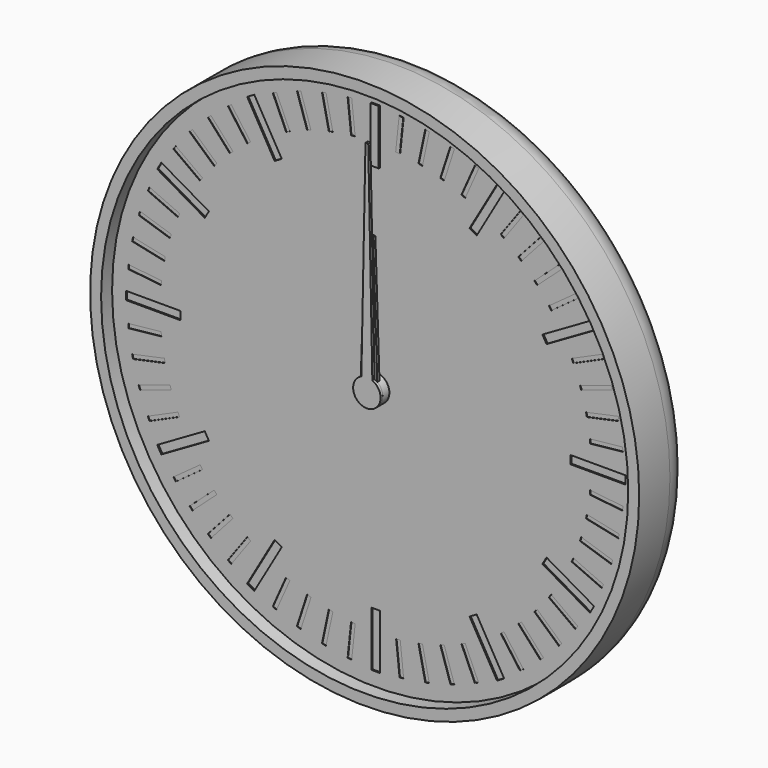
from build123d import *

# Parameters (mm, degrees)
F0_R      = 100
F1_DEPTH  = 24
F2_R      = 10
F3_T      = -4
F4_R      = 5
F4_R_2    = 3
F5_DEPTH  = 2
F6_DEPTH  = 19
F7_DEPTH  = 8
F9_DEPTH  = 4
F11_DEPTH = 4
F12_R     = 5
F12_R_2   = 3
F13_DEPTH = 2
F14_R     = 3
F15_DEPTH = 4
F17_DEPTH = 4
F18_R     = 3
F19_DEPTH = 2
F20_R     = 98
F20_R_2   = 5
F21_DEPTH = 1
F23_R     = 5
F23_R_2   = 3
F24_DEPTH = 2
F25_W     = 3
F25_H     = 20
F25_W_2   = 20
F25_H_2   = 3
F26_DEPTH = 0.5
F27_W     = 1.5
F27_H     = 12
F27_W_2   = 12
F27_H_2   = 1.5
F28_DEPTH = 0.2
F29_DEPTH = 1
F30_DEPTH = 0.4
F31_R     = 5
F31_R_2   = 3
F32_DEPTH = 5
F33_R     = 3
F34_DEPTH = 1
F36_DEPTH = 1


with BuildPart() as f1:
    # F0 (on Front) → F1 (new body)
    with BuildSketch(Plane.XZ):
        Circle(F0_R)
    extrude(amount=F1_DEPTH)

    # F2
    f2_edges = [f1.edges().sort_by_distance(p)[0] for p in [
        (-100, 0, 0),
    ]]
    fillet(f2_edges, radius=F2_R)

    # F3
    f3_openings = [f1.faces().sort_by_distance(p)[0] for p in [
        (0, -24, 0),
    ]]
    offset(amount=F3_T, openings=f3_openings)

    # F4 (on face) → F5 (join)
    with BuildSketch(Plane.XZ.offset(4)):
        Circle(F4_R)
        Circle(F4_R_2, mode=Mode.SUBTRACT)
        with Locations((40, 0)):
            Circle(F4_R)
        with Locations((40, 0)):
            Circle(F4_R_2, mode=Mode.SUBTRACT)
    extrude(amount=F5_DEPTH)


with BuildPart() as f6:
    # F6 (new): a face of the model
    f6_faces = [f1.part.faces().sort_by_distance(p)[0] for p in [
        (0, -4, 0),
    ]]
    extrude(f6_faces, amount=F6_DEPTH)

    # F8 (on face) → F9 (join)
    with BuildSketch(Plane.XZ.offset(6)):
        with BuildLine():
            ThreePointArc((9.2729637667, -1.3794085621), (9.3494561423, -0.6915886375), (9.375, 0))
            ThreePointArc((9.375, 0), (9.3494561423, 0.6915886375), (9.2729637667, 1.3794085621))
            ThreePointArc((9.2729637667, 1.3794085621), (8.9161548403, 2.8970343223), (8.3127812852, 4.3345463782))
            ThreePointArc((8.3127812852, 4.3345463782), (7.5845343223, 5.5104867402), (6.6911892658, 6.566476316))
            ThreePointArc((6.6911892658, 6.566476316), (5.5104867402, 7.5845343223), (4.1773988938, 8.3928519278))
            ThreePointArc((4.1773988938, 8.3928519278), (2.8970343223, 8.9161548403), (1.5536078905, 9.2453733036))
            ThreePointArc((1.5536078905, 9.2453733036), (0, 9.375), (-1.5536078905, 9.2453733036))
            ThreePointArc((-1.5536078905, 9.2453733036), (-2.8970343223, 8.9161548403), (-4.1773988938, 8.3928519278))
            ThreePointArc((-4.1773988938, 8.3928519278), (-5.5104867402, 7.5845343223), (-6.6911892658, 6.566476316))
            ThreePointArc((-6.6911892658, 6.566476316), (-7.5845343223, 5.5104867402), (-8.3127812852, 4.3345463782))
            ThreePointArc((-8.3127812852, 4.3345463782), (-8.9161548403, 2.8970343223), (-9.2729637667, 1.3794085621))
            ThreePointArc((-9.2729637667, 1.3794085621), (-9.375, 0), (-9.2729637667, -1.3794085621))
            ThreePointArc((-9.2729637667, -1.3794085621), (-8.9161548403, -2.8970343223), (-8.3127812852, -4.3345463782))
            ThreePointArc((-8.3127812852, -4.3345463782), (-7.5845343223, -5.5104867402), (-6.6911892658, -6.566476316))
            ThreePointArc((-6.6911892658, -6.566476316), (-5.5104867402, -7.5845343223), (-4.1773988938, -8.3928519278))
            ThreePointArc((-4.1773988938, -8.3928519278), (-2.8970343223, -8.9161548403), (-1.5536078905, -9.2453733036))
            ThreePointArc((-1.5536078905, -9.2453733036), (0, -9.375), (1.5536078905, -9.2453733036))
            ThreePointArc((1.5536078905, -9.2453733036), (2.8970343223, -8.9161548403), (4.1773988938, -8.3928519278))
            ThreePointArc((4.1773988938, -8.3928519278), (5.5104867402, -7.5845343223), (6.6911892658, -6.566476316))
            ThreePointArc((6.6911892658, -6.566476316), (7.5845343223, -5.5104867402), (8.3127812852, -4.3345463782))
            ThreePointArc((8.3127812852, -4.3345463782), (8.9161548403, -2.8970343223), (9.2729637667, -1.3794085621))
        make_face()
        with BuildLine():
            ThreePointArc((8.3127812852, 4.3345463782), (8.9161548403, 2.8970343223), (9.2729637667, 1.3794085621))
            Line((9.2729637667, 1.3794085621), (11.1823199426, 2.3946312492))
            Line((11.1823199426, 2.3946312492), (10.8182678729, 3.515068311))
            Line((10.8182678729, 3.515068311), (10.4542158031, 4.6355053728))
            Line((10.4542158031, 4.6355053728), (8.3127812852, 4.3345463782))
        make_face()
        with BuildLine():
            Line((11.1823199426, -2.3946312492), (9.2729637667, -1.3794085621))
            ThreePointArc((9.2729637667, -1.3794085621), (8.9161548403, -2.8970343223), (8.3127812852, -4.3345463782))
            Line((8.3127812852, -4.3345463782), (10.4542158031, -4.6355053728))
            Line((10.4542158031, -4.6355053728), (10.8182678729, -3.515068311))
            Line((10.8182678729, -3.515068311), (11.1823199426, -2.3946312492))
        make_face()
        with BuildLine():
            ThreePointArc((4.1773988938, 8.3928519278), (5.5104867402, 7.5845343223), (6.6911892658, 6.566476316))
            Line((6.6911892658, 6.566476316), (7.6391579371, 8.5101001246))
            Line((7.6391579371, 8.5101001246), (6.6860572448, 9.202568311))
            Line((6.6860572448, 9.202568311), (5.7329565525, 9.8950364974))
            Line((5.7329565525, 9.8950364974), (4.1773988938, 8.3928519278))
        make_face()
        with BuildLine():
            Line((7.6391579371, -8.5101001246), (6.6911892658, -6.566476316))
            ThreePointArc((6.6911892658, -6.566476316), (5.5104867402, -7.5845343223), (4.1773988938, -8.3928519278))
            Line((4.1773988938, -8.3928519278), (5.7329565525, -9.8950364974))
            Line((5.7329565525, -9.8950364974), (6.6860572448, -9.202568311))
            Line((6.6860572448, -9.202568311), (7.6391579371, -8.5101001246))
        make_face()
        with BuildLine():
            ThreePointArc((-1.5536078905, 9.2453733036), (0, 9.375), (1.5536078905, 9.2453733036))
            Line((1.5536078905, 9.2453733036), (1.1780972451, 11.375))
            Line((1.1780972451, 11.375), (0, 11.375))
            Line((0, 11.375), (-1.1780972451, 11.375))
            Line((-1.1780972451, 11.375), (-1.5536078905, 9.2453733036))
        make_face()
        with BuildLine():
            Line((1.1780972451, -11.375), (1.5536078905, -9.2453733036))
            ThreePointArc((1.5536078905, -9.2453733036), (0, -9.375), (-1.5536078905, -9.2453733036))
            Line((-1.5536078905, -9.2453733036), (-1.1780972451, -11.375))
            Line((-1.1780972451, -11.375), (0, -11.375))
            Line((0, -11.375), (1.1780972451, -11.375))
        make_face()
        with BuildLine():
            ThreePointArc((-6.6911892658, 6.566476316), (-5.5104867402, 7.5845343223), (-4.1773988938, 8.3928519278))
            Line((-4.1773988938, 8.3928519278), (-5.7329565525, 9.8950364974))
            Line((-5.7329565525, 9.8950364974), (-6.6860572448, 9.202568311))
            Line((-6.6860572448, 9.202568311), (-7.6391579371, 8.5101001246))
            Line((-7.6391579371, 8.5101001246), (-6.6911892658, 6.566476316))
        make_face()
        with BuildLine():
            Line((-5.7329565525, -9.8950364974), (-4.1773988938, -8.3928519278))
            ThreePointArc((-4.1773988938, -8.3928519278), (-5.5104867402, -7.5845343223), (-6.6911892658, -6.566476316))
            Line((-6.6911892658, -6.566476316), (-7.6391579371, -8.5101001246))
            Line((-7.6391579371, -8.5101001246), (-6.6860572448, -9.202568311))
            Line((-6.6860572448, -9.202568311), (-5.7329565525, -9.8950364974))
        make_face()
        with BuildLine():
            ThreePointArc((-9.2729637667, 1.3794085621), (-8.9161548403, 2.8970343223), (-8.3127812852, 4.3345463782))
            Line((-8.3127812852, 4.3345463782), (-10.4542158031, 4.6355053728))
            Line((-10.4542158031, 4.6355053728), (-10.8182678729, 3.515068311))
            Line((-10.8182678729, 3.515068311), (-11.1823199426, 2.3946312492))
            Line((-11.1823199426, 2.3946312492), (-9.2729637667, 1.3794085621))
        make_face()
        with BuildLine():
            Line((-10.4542158031, -4.6355053728), (-8.3127812852, -4.3345463782))
            ThreePointArc((-8.3127812852, -4.3345463782), (-8.9161548403, -2.8970343223), (-9.2729637667, -1.3794085621))
            Line((-9.2729637667, -1.3794085621), (-11.1823199426, -2.3946312492))
            Line((-11.1823199426, -2.3946312492), (-10.8182678729, -3.515068311))
            Line((-10.8182678729, -3.515068311), (-10.4542158031, -4.6355053728))
        make_face()
    extrude(amount=F9_DEPTH)

    # F35 (on face) → F36 (join)
    with BuildSketch(Plane.XZ.offset(23)):
        with BuildLine():
            ThreePointArc((-2, 4.582575695), (-2.7386127875, -4.1833001327), (5, 0))
            ThreePointArc((5, 0), (4.1833001327, 2.7386127875), (2, 4.582575695))
            ThreePointArc((2, 4.582575695), (0, 5), (-2, 4.582575695))
        make_face()
        with BuildLine():
            ThreePointArc((-2, 4.582575695), (0, 5), (2, 4.582575695))
            Line((2, 4.582575695), (0.5, 80))
            Line((0.5, 80), (0, 80))
            Line((0, 80), (-0.5, 80))
            Line((-0.5, 80), (-2, 4.582575695))
        make_face()
    extrude(amount=-F36_DEPTH)


with BuildPart() as f7:
    # F7 (new): a face of the model
    f7_faces = [f1.part.faces().sort_by_distance(p)[0] for p in [
        (40, -4, 0),
    ]]
    extrude(f7_faces, amount=F7_DEPTH)

    # F10 (on face) → F11 (join)
    with BuildSketch(Plane.XZ.offset(6)):
        with BuildLine():
            ThreePointArc((68.0829066802, -1.5381733945), (68.1144747006, -0.7693746225), (68.125, 0))
            ThreePointArc((68.125, 0), (68.1144747006, 0.7693746225), (68.0829066802, 1.5381733945))
            ThreePointArc((68.0829066802, 1.5381733945), (67.9709283072, 2.9398630294), (67.7890320221, 4.3342039956))
            ThreePointArc((67.7890320221, 4.3342039956), (67.5104012706, 5.8475163042), (67.1494235596, 7.3433252263))
            ThreePointArc((67.1494235596, 7.3433252263), (66.7484645208, 8.6911029668), (66.280643318, 10.0171558733))
            ThreePointArc((66.280643318, 10.0171558733), (65.6934659962, 11.4394680865), (65.0293803521, 12.8275385085))
            ThreePointArc((65.0293803521, 12.8275385085), (64.3569644814, 14.0625), (63.6236643925, 15.2623099717))
            ThreePointArc((63.6236643925, 15.2623099717), (62.7536029668, 16.5314602207), (61.815433119, 17.7511268046))
            ThreePointArc((61.815433119, 17.7511268046), (60.9009482166, 18.8192983038), (59.934217974, 19.8404278876))
            ThreePointArc((59.934217974, 19.8404278876), (58.8192983038, 20.9009482166), (57.6480467764, 21.8989056799))
            ThreePointArc((57.6480467764, 21.8989056799), (56.5314602207, 22.7536029668), (55.3735505752, 23.5514238999))
            ThreePointArc((55.3735505752, 23.5514238999), (54.0625, 24.3569644814), (52.709356105, 25.0895972944))
            ThreePointArc((52.709356105, 25.0895972944), (51.4394680865, 25.6934659962), (50.1409852457, 26.2331096755))
            ThreePointArc((50.1409852457, 26.2331096755), (48.6911029668, 26.7484645208), (47.2152055856, 27.1837531139))
            ThreePointArc((47.2152055856, 27.1837531139), (45.8475163042, 27.5104012706), (44.4652101991, 27.7682826779))
            ThreePointArc((44.4652101991, 27.7682826779), (42.9398630294, 27.9709283072), (41.4057159597, 28.0898484802))
            ThreePointArc((41.4057159597, 28.0898484802), (40, 28.125), (38.5942840403, 28.0898484802))
            ThreePointArc((38.5942840403, 28.0898484802), (37.0601369706, 27.9709283072), (35.5347898009, 27.7682826779))
            ThreePointArc((35.5347898009, 27.7682826779), (34.1524836958, 27.5104012706), (32.7847944144, 27.1837531139))
            ThreePointArc((32.7847944144, 27.1837531139), (31.3088970332, 26.7484645208), (29.8590147543, 26.2331096755))
            ThreePointArc((29.8590147543, 26.2331096755), (28.5605319135, 25.6934659962), (27.290643895, 25.0895972944))
            ThreePointArc((27.290643895, 25.0895972944), (25.9375, 24.3569644814), (24.6264494248, 23.5514238999))
            ThreePointArc((24.6264494248, 23.5514238999), (23.4685397793, 22.7536029668), (22.3519532236, 21.8989056799))
            ThreePointArc((22.3519532236, 21.8989056799), (21.1807016962, 20.9009482166), (20.065782026, 19.8404278876))
            ThreePointArc((20.065782026, 19.8404278876), (19.0990517834, 18.8192983038), (18.184566881, 17.7511268046))
            ThreePointArc((18.184566881, 17.7511268046), (17.2463970332, 16.5314602207), (16.3763356075, 15.2623099717))
            ThreePointArc((16.3763356075, 15.2623099717), (15.6430355186, 14.0625), (14.9706196479, 12.8275385085))
            ThreePointArc((14.9706196479, 12.8275385085), (14.3065340038, 11.4394680865), (13.719356682, 10.0171558733))
            ThreePointArc((13.719356682, 10.0171558733), (13.2515354792, 8.6911029668), (12.8505764404, 7.3433252263))
            ThreePointArc((12.8505764404, 7.3433252263), (12.4895987294, 5.8475163042), (12.2109679779, 4.3342039956))
            ThreePointArc((12.2109679779, 4.3342039956), (12.0290716928, 2.9398630294), (11.9170933198, 1.5381733945))
            ThreePointArc((11.9170933198, 1.5381733945), (11.875, 0), (11.9170933198, -1.5381733945))
            ThreePointArc((11.9170933198, -1.5381733945), (12.0290716928, -2.9398630294), (12.2109679779, -4.3342039956))
            ThreePointArc((12.2109679779, -4.3342039956), (12.4895987294, -5.8475163042), (12.8505764404, -7.3433252263))
            ThreePointArc((12.8505764404, -7.3433252263), (13.2515354792, -8.6911029668), (13.719356682, -10.0171558733))
            ThreePointArc((13.719356682, -10.0171558733), (14.3065340038, -11.4394680865), (14.9706196479, -12.8275385085))
            ThreePointArc((14.9706196479, -12.8275385085), (15.6430355186, -14.0625), (16.3763356075, -15.2623099717))
            ThreePointArc((16.3763356075, -15.2623099717), (17.2463970332, -16.5314602207), (18.184566881, -17.7511268046))
            ThreePointArc((18.184566881, -17.7511268046), (19.0990517834, -18.8192983038), (20.065782026, -19.8404278876))
            ThreePointArc((20.065782026, -19.8404278876), (21.1807016962, -20.9009482166), (22.3519532236, -21.8989056799))
            ThreePointArc((22.3519532236, -21.8989056799), (23.4685397793, -22.7536029668), (24.6264494248, -23.5514238999))
            ThreePointArc((24.6264494248, -23.5514238999), (25.9375, -24.3569644814), (27.290643895, -25.0895972944))
            ThreePointArc((27.290643895, -25.0895972944), (28.5605319135, -25.6934659962), (29.8590147543, -26.2331096755))
            ThreePointArc((29.8590147543, -26.2331096755), (31.3088970332, -26.7484645208), (32.7847944144, -27.1837531139))
            ThreePointArc((32.7847944144, -27.1837531139), (34.1524836958, -27.5104012706), (35.5347898009, -27.7682826779))
            ThreePointArc((35.5347898009, -27.7682826779), (37.0601369706, -27.9709283072), (38.5942840403, -28.0898484802))
            ThreePointArc((38.5942840403, -28.0898484802), (40, -28.125), (41.4057159597, -28.0898484802))
            ThreePointArc((41.4057159597, -28.0898484802), (42.9398630294, -27.9709283072), (44.4652101991, -27.7682826779))
            ThreePointArc((44.4652101991, -27.7682826779), (45.8475163042, -27.5104012706), (47.2152055856, -27.1837531139))
            ThreePointArc((47.2152055856, -27.1837531139), (48.6911029668, -26.7484645208), (50.1409852457, -26.2331096755))
            ThreePointArc((50.1409852457, -26.2331096755), (51.4394680865, -25.6934659962), (52.709356105, -25.0895972944))
            ThreePointArc((52.709356105, -25.0895972944), (54.0625, -24.3569644814), (55.3735505752, -23.5514238999))
            ThreePointArc((55.3735505752, -23.5514238999), (56.5314602207, -22.7536029668), (57.6480467764, -21.8989056799))
            ThreePointArc((57.6480467764, -21.8989056799), (58.8192983038, -20.9009482166), (59.934217974, -19.8404278876))
            ThreePointArc((59.934217974, -19.8404278876), (60.9009482166, -18.8192983038), (61.815433119, -17.7511268046))
            ThreePointArc((61.815433119, -17.7511268046), (62.7536029668, -16.5314602207), (63.6236643925, -15.2623099717))
            ThreePointArc((63.6236643925, -15.2623099717), (64.3569644814, -14.0625), (65.0293803521, -12.8275385085))
            ThreePointArc((65.0293803521, -12.8275385085), (65.6934659962, -11.4394680865), (66.280643318, -10.0171558733))
            ThreePointArc((66.280643318, -10.0171558733), (66.7484645208, -8.6911029668), (67.1494235596, -7.3433252263))
            ThreePointArc((67.1494235596, -7.3433252263), (67.5104012706, -5.8475163042), (67.7890320221, -4.3342039956))
            ThreePointArc((67.7890320221, -4.3342039956), (67.9709283072, -2.9398630294), (68.0829066802, -1.5381733945))
        make_face()
        with BuildLine():
            ThreePointArc((68.0829066802, 1.5381733945), (68.1144747006, 0.7693746225), (68.125, 0))
            ThreePointArc((68.125, 0), (68.1144747006, -0.7693746225), (68.0829066802, -1.5381733945))
            Line((68.0829066802, -1.5381733945), (70.125, -1.1780972451))
            Line((70.125, -1.1780972451), (70.125, 0))
            Line((70.125, 0), (70.125, 1.1780972451))
            Line((70.125, 1.1780972451), (68.0829066802, 1.5381733945))
        make_face()
        with BuildLine():
            ThreePointArc((67.1494235596, 7.3433252263), (67.5104012706, 5.8475163042), (67.7890320221, 4.3342039956))
            Line((67.7890320221, 4.3342039956), (69.7116366623, 5.1109866922))
            Line((69.7116366623, 5.1109866922), (69.4666964721, 6.2633396859))
            Line((69.4666964721, 6.2633396859), (69.2217562819, 7.4156926796))
            Line((69.2217562819, 7.4156926796), (67.1494235596, 7.3433252263))
        make_face()
        with BuildLine():
            Line((69.7116366623, -5.1109866922), (67.7890320221, -4.3342039956))
            ThreePointArc((67.7890320221, -4.3342039956), (67.5104012706, -5.8475163042), (67.1494235596, -7.3433252263))
            Line((67.1494235596, -7.3433252263), (69.2217562819, -7.4156926796))
            Line((69.2217562819, -7.4156926796), (69.4666964721, -6.2633396859))
            Line((69.4666964721, -6.2633396859), (69.7116366623, -5.1109866922))
        make_face()
        with BuildLine():
            ThreePointArc((65.0293803521, 12.8275385085), (65.6934659962, 11.4394680865), (66.280643318, 10.0171558733))
            Line((66.280643318, 10.0171558733), (67.9997322302, 11.1766959857))
            Line((67.9997322302, 11.1766959857), (67.5205569115, 12.2529413727))
            Line((67.5205569115, 12.2529413727), (67.0413815928, 13.3291867596))
            Line((67.0413815928, 13.3291867596), (65.0293803521, 12.8275385085))
        make_face()
        with BuildLine():
            Line((67.9997322302, -11.1766959857), (66.280643318, -10.0171558733))
            ThreePointArc((66.280643318, -10.0171558733), (65.6934659962, -11.4394680865), (65.0293803521, -12.8275385085))
            Line((65.0293803521, -12.8275385085), (67.0413815928, -13.3291867596))
            Line((67.0413815928, -13.3291867596), (67.5205569115, -12.2529413727))
            Line((67.5205569115, -12.2529413727), (67.9997322302, -11.1766959857))
        make_face()
        with BuildLine():
            ThreePointArc((61.815433119, 17.7511268046), (62.7536029668, 16.5314602207), (63.6236643925, 15.2623099717))
            Line((63.6236643925, 15.2623099717), (65.064105142, 16.753930033))
            Line((65.064105142, 16.753930033), (64.3716369555, 17.7070307253))
            Line((64.3716369555, 17.7070307253), (63.6791687691, 18.6601314176))
            Line((63.6791687691, 18.6601314176), (61.815433119, 17.7511268046))
        make_face()
        with BuildLine():
            Line((65.064105142, -16.753930033), (63.6236643925, -15.2623099717))
            ThreePointArc((63.6236643925, -15.2623099717), (62.7536029668, -16.5314602207), (61.815433119, -17.7511268046))
            Line((61.815433119, -17.7511268046), (63.6791687691, -18.6601314176))
            Line((63.6791687691, -18.6601314176), (64.3716369555, -17.7070307253))
            Line((64.3716369555, -17.7070307253), (65.064105142, -16.753930033))
        make_face()
        with BuildLine():
            ThreePointArc((57.6480467764, 21.8989056799), (58.8192983038, 20.9009482166), (59.934217974, 19.8404278876))
            Line((59.934217974, 19.8404278876), (61.0330563882, 21.5989369435))
            Line((61.0330563882, 21.5989369435), (60.1575595166, 22.3872378675))
            Line((60.1575595166, 22.3872378675), (59.282062645, 23.1755387915))
            Line((59.282062645, 23.1755387915), (57.6480467764, 21.8989056799))
        make_face()
        with BuildLine():
            Line((61.0330563882, -21.5989369435), (59.934217974, -19.8404278876))
            ThreePointArc((59.934217974, -19.8404278876), (58.8192983038, -20.9009482166), (57.6480467764, -21.8989056799))
            Line((57.6480467764, -21.8989056799), (59.282062645, -23.1755387915))
            Line((59.282062645, -23.1755387915), (60.1575595166, -22.3872378675))
            Line((60.1575595166, -22.3872378675), (61.0330563882, -21.5989369435))
        make_face()
        with BuildLine():
            ThreePointArc((52.709356105, 25.0895972944), (54.0625, 24.3569644814), (55.3735505752, 23.5514238999))
            Line((55.3735505752, 23.5514238999), (56.0827621424, 25.4999666665))
            Line((56.0827621424, 25.4999666665), (55.0625, 26.089015289))
            Line((55.0625, 26.089015289), (54.0422378576, 26.6780639116))
            Line((54.0422378576, 26.6780639116), (52.709356105, 25.0895972944))
        make_face()
        with BuildLine():
            Line((56.0827621424, -25.4999666665), (55.3735505752, -23.5514238999))
            ThreePointArc((55.3735505752, -23.5514238999), (54.0625, -24.3569644814), (52.709356105, -25.0895972944))
            Line((52.709356105, -25.0895972944), (54.0422378576, -26.6780639116))
            Line((54.0422378576, -26.6780639116), (55.0625, -26.089015289))
            Line((55.0625, -26.089015289), (56.0827621424, -25.4999666665))
        make_face()
        with BuildLine():
            ThreePointArc((47.2152055856, 27.1837531139), (48.6911029668, 26.7484645208), (50.1409852457, 26.2331096755))
            Line((50.1409852457, 26.2331096755), (50.4295740173, 28.2865254836))
            Line((50.4295740173, 28.2865254836), (49.3091369555, 28.6505775534))
            Line((49.3091369555, 28.6505775534), (48.1886998938, 29.0146296232))
            Line((48.1886998938, 29.0146296232), (47.2152055856, 27.1837531139))
        make_face()
        with BuildLine():
            Line((50.4295740173, -28.2865254836), (50.1409852457, -26.2331096755))
            ThreePointArc((50.1409852457, -26.2331096755), (48.6911029668, -26.7484645208), (47.2152055856, -27.1837531139))
            Line((47.2152055856, -27.1837531139), (48.1886998938, -29.0146296232))
            Line((48.1886998938, -29.0146296232), (49.3091369555, -28.6505775534))
            Line((49.3091369555, -28.6505775534), (50.4295740173, -28.2865254836))
        make_face()
        with BuildLine():
            ThreePointArc((41.4057159597, 28.0898484802), (42.9398630294, 27.9709283072), (44.4652101991, 27.7682826779))
            Line((44.4652101991, 27.7682826779), (44.3205634611, 29.8368274034))
            Line((44.3205634611, 29.8368274034), (43.1489199559, 29.959972098))
            Line((43.1489199559, 29.959972098), (41.9772764508, 30.0831167926))
            Line((41.9772764508, 30.0831167926), (41.4057159597, 28.0898484802))
        make_face()
        with BuildLine():
            Line((44.3205634611, -29.8368274034), (44.4652101991, -27.7682826779))
            ThreePointArc((44.4652101991, -27.7682826779), (42.9398630294, -27.9709283072), (41.4057159597, -28.0898484802))
            Line((41.4057159597, -28.0898484802), (41.9772764508, -30.0831167926))
            Line((41.9772764508, -30.0831167926), (43.1489199559, -29.959972098))
            Line((43.1489199559, -29.959972098), (44.3205634611, -29.8368274034))
        make_face()
        with BuildLine():
            ThreePointArc((35.5347898009, 27.7682826779), (37.0601369706, 27.9709283072), (38.5942840403, 28.0898484802))
            Line((38.5942840403, 28.0898484802), (38.0227235492, 30.0831167926))
            Line((38.0227235492, 30.0831167926), (36.8510800441, 29.959972098))
            Line((36.8510800441, 29.959972098), (35.6794365389, 29.8368274034))
            Line((35.6794365389, 29.8368274034), (35.5347898009, 27.7682826779))
        make_face()
        with BuildLine():
            Line((38.0227235492, -30.0831167926), (38.5942840403, -28.0898484802))
            ThreePointArc((38.5942840403, -28.0898484802), (37.0601369706, -27.9709283072), (35.5347898009, -27.7682826779))
            Line((35.5347898009, -27.7682826779), (35.6794365389, -29.8368274034))
            Line((35.6794365389, -29.8368274034), (36.8510800441, -29.959972098))
            Line((36.8510800441, -29.959972098), (38.0227235492, -30.0831167926))
        make_face()
        with BuildLine():
            ThreePointArc((29.8590147543, 26.2331096755), (31.3088970332, 26.7484645208), (32.7847944144, 27.1837531139))
            Line((32.7847944144, 27.1837531139), (31.8113001062, 29.0146296232))
            Line((31.8113001062, 29.0146296232), (30.6908630445, 28.6505775534))
            Line((30.6908630445, 28.6505775534), (29.5704259827, 28.2865254836))
            Line((29.5704259827, 28.2865254836), (29.8590147543, 26.2331096755))
        make_face()
        with BuildLine():
            Line((31.8113001062, -29.0146296232), (32.7847944144, -27.1837531139))
            ThreePointArc((32.7847944144, -27.1837531139), (31.3088970332, -26.7484645208), (29.8590147543, -26.2331096755))
            Line((29.8590147543, -26.2331096755), (29.5704259827, -28.2865254836))
            Line((29.5704259827, -28.2865254836), (30.6908630445, -28.6505775534))
            Line((30.6908630445, -28.6505775534), (31.8113001062, -29.0146296232))
        make_face()
        with BuildLine():
            ThreePointArc((24.6264494248, 23.5514238999), (25.9375, 24.3569644814), (27.290643895, 25.0895972944))
            Line((27.290643895, 25.0895972944), (25.9577621424, 26.6780639116))
            Line((25.9577621424, 26.6780639116), (24.9375, 26.089015289))
            Line((24.9375, 26.089015289), (23.9172378576, 25.4999666665))
            Line((23.9172378576, 25.4999666665), (24.6264494248, 23.5514238999))
        make_face()
        with BuildLine():
            Line((25.9577621424, -26.6780639116), (27.290643895, -25.0895972944))
            ThreePointArc((27.290643895, -25.0895972944), (25.9375, -24.3569644814), (24.6264494248, -23.5514238999))
            Line((24.6264494248, -23.5514238999), (23.9172378576, -25.4999666665))
            Line((23.9172378576, -25.4999666665), (24.9375, -26.089015289))
            Line((24.9375, -26.089015289), (25.9577621424, -26.6780639116))
        make_face()
        with BuildLine():
            ThreePointArc((20.065782026, 19.8404278876), (21.1807016962, 20.9009482166), (22.3519532236, 21.8989056799))
            Line((22.3519532236, 21.8989056799), (20.717937355, 23.1755387915))
            Line((20.717937355, 23.1755387915), (19.8424404834, 22.3872378675))
            Line((19.8424404834, 22.3872378675), (18.9669436118, 21.5989369435))
            Line((18.9669436118, 21.5989369435), (20.065782026, 19.8404278876))
        make_face()
        with BuildLine():
            Line((20.717937355, -23.1755387915), (22.3519532236, -21.8989056799))
            ThreePointArc((22.3519532236, -21.8989056799), (21.1807016962, -20.9009482166), (20.065782026, -19.8404278876))
            Line((20.065782026, -19.8404278876), (18.9669436118, -21.5989369435))
            Line((18.9669436118, -21.5989369435), (19.8424404834, -22.3872378675))
            Line((19.8424404834, -22.3872378675), (20.717937355, -23.1755387915))
        make_face()
        with BuildLine():
            ThreePointArc((16.3763356075, 15.2623099717), (17.2463970332, 16.5314602207), (18.184566881, 17.7511268046))
            Line((18.184566881, 17.7511268046), (16.3208312309, 18.6601314176))
            Line((16.3208312309, 18.6601314176), (15.6283630445, 17.7070307253))
            Line((15.6283630445, 17.7070307253), (14.935894858, 16.753930033))
            Line((14.935894858, 16.753930033), (16.3763356075, 15.2623099717))
        make_face()
        with BuildLine():
            Line((16.3208312309, -18.6601314176), (18.184566881, -17.7511268046))
            ThreePointArc((18.184566881, -17.7511268046), (17.2463970332, -16.5314602207), (16.3763356075, -15.2623099717))
            Line((16.3763356075, -15.2623099717), (14.935894858, -16.753930033))
            Line((14.935894858, -16.753930033), (15.6283630445, -17.7070307253))
            Line((15.6283630445, -17.7070307253), (16.3208312309, -18.6601314176))
        make_face()
        with BuildLine():
            ThreePointArc((13.719356682, 10.0171558733), (14.3065340038, 11.4394680865), (14.9706196479, 12.8275385085))
            Line((14.9706196479, 12.8275385085), (12.9586184072, 13.3291867596))
            Line((12.9586184072, 13.3291867596), (12.4794430885, 12.2529413727))
            Line((12.4794430885, 12.2529413727), (12.0002677698, 11.1766959857))
            Line((12.0002677698, 11.1766959857), (13.719356682, 10.0171558733))
        make_face()
        with BuildLine():
            Line((12.9586184072, -13.3291867596), (14.9706196479, -12.8275385085))
            ThreePointArc((14.9706196479, -12.8275385085), (14.3065340038, -11.4394680865), (13.719356682, -10.0171558733))
            Line((13.719356682, -10.0171558733), (12.0002677698, -11.1766959857))
            Line((12.0002677698, -11.1766959857), (12.4794430885, -12.2529413727))
            Line((12.4794430885, -12.2529413727), (12.9586184072, -13.3291867596))
        make_face()
        with BuildLine():
            ThreePointArc((12.2109679779, 4.3342039956), (12.4895987294, 5.8475163042), (12.8505764404, 7.3433252263))
            Line((12.8505764404, 7.3433252263), (10.7782437181, 7.4156926796))
            Line((10.7782437181, 7.4156926796), (10.5333035279, 6.2633396859))
            Line((10.5333035279, 6.2633396859), (10.2883633377, 5.1109866922))
            Line((10.2883633377, 5.1109866922), (12.2109679779, 4.3342039956))
        make_face()
        with BuildLine():
            Line((10.7782437181, -7.4156926796), (12.8505764404, -7.3433252263))
            ThreePointArc((12.8505764404, -7.3433252263), (12.4895987294, -5.8475163042), (12.2109679779, -4.3342039956))
            Line((12.2109679779, -4.3342039956), (10.2883633377, -5.1109866922))
            Line((10.2883633377, -5.1109866922), (10.5333035279, -6.2633396859))
            Line((10.5333035279, -6.2633396859), (10.7782437181, -7.4156926796))
        make_face()
        with BuildLine():
            ThreePointArc((11.9170933198, -1.5381733945), (11.875, 0), (11.9170933198, 1.5381733945))
            Line((11.9170933198, 1.5381733945), (9.875, 1.1780972451))
            Line((9.875, 1.1780972451), (9.875, 0))
            Line((9.875, 0), (9.875, -1.1780972451))
            Line((9.875, -1.1780972451), (11.9170933198, -1.5381733945))
        make_face()
    extrude(amount=F11_DEPTH)

    # F16 (on face) → F17 (join)
    with BuildSketch(Plane.XZ.offset(12)):
        with BuildLine():
            ThreePointArc((47.4288750323, -1.0304444454), (47.4821976298, -0.5164480894), (47.5, 0))
            ThreePointArc((47.5, 0), (47.4821976298, 0.5164480894), (47.4288750323, 1.0304444454))
            ThreePointArc((47.4288750323, 1.0304444454), (47.1329238722, 2.3176274578), (46.6157661985, 3.532936117))
            ThreePointArc((46.6157661985, 3.532936117), (46.0676274578, 4.4083893922), (45.4044061018, 5.2002302532))
            ThreePointArc((45.4044061018, 5.2002302532), (44.4083893922, 6.0676274578), (43.2756595386, 6.7468551628))
            ThreePointArc((43.2756595386, 6.7468551628), (42.3176274578, 7.1329238722), (41.3156377295, 7.3837048536))
            ThreePointArc((41.3156377295, 7.3837048536), (40, 7.5), (38.6843622705, 7.3837048536))
            ThreePointArc((38.6843622705, 7.3837048536), (37.6823725422, 7.1329238722), (36.7243404614, 6.7468551628))
            ThreePointArc((36.7243404614, 6.7468551628), (35.5916106078, 6.0676274578), (34.5955938982, 5.2002302532))
            ThreePointArc((34.5955938982, 5.2002302532), (33.9323725422, 4.4083893922), (33.3842338015, 3.532936117))
            ThreePointArc((33.3842338015, 3.532936117), (32.8670761278, 2.3176274578), (32.5711249677, 1.0304444454))
            ThreePointArc((32.5711249677, 1.0304444454), (32.5, 0), (32.5711249677, -1.0304444454))
            ThreePointArc((32.5711249677, -1.0304444454), (32.8670761278, -2.3176274578), (33.3842338015, -3.532936117))
            ThreePointArc((33.3842338015, -3.532936117), (33.9323725422, -4.4083893922), (34.5955938982, -5.2002302532))
            ThreePointArc((34.5955938982, -5.2002302532), (35.5916106078, -6.0676274578), (36.7243404614, -6.7468551628))
            ThreePointArc((36.7243404614, -6.7468551628), (37.6823725422, -7.1329238722), (38.6843622705, -7.3837048536))
            ThreePointArc((38.6843622705, -7.3837048536), (40, -7.5), (41.3156377295, -7.3837048536))
            ThreePointArc((41.3156377295, -7.3837048536), (42.3176274578, -7.1329238722), (43.2756595386, -6.7468551628))
            ThreePointArc((43.2756595386, -6.7468551628), (44.4083893922, -6.0676274578), (45.4044061018, -5.2002302532))
            ThreePointArc((45.4044061018, -5.2002302532), (46.0676274578, -4.4083893922), (46.6157661985, -3.532936117))
            ThreePointArc((46.6157661985, -3.532936117), (47.1329238722, -2.3176274578), (47.4288750323, -1.0304444454))
        make_face()
        with BuildLine():
            ThreePointArc((46.6157661985, 3.532936117), (47.1329238722, 2.3176274578), (47.4288750323, 1.0304444454))
            Line((47.4288750323, 1.0304444454), (49.3262785606, 2.0393117971))
            Line((49.3262785606, 2.0393117971), (48.743795249, 3.832011096))
            Line((48.743795249, 3.832011096), (46.6157661985, 3.532936117))
        make_face()
        with BuildLine():
            Line((49.3262785606, -2.0393117971), (47.4288750323, -1.0304444454))
            ThreePointArc((47.4288750323, -1.0304444454), (47.1329238722, -2.3176274578), (46.6157661985, -3.532936117))
            Line((46.6157661985, -3.532936117), (48.743795249, -3.832011096))
            Line((48.743795249, -3.832011096), (49.3262785606, -2.0393117971))
        make_face()
        with BuildLine():
            ThreePointArc((43.2756595386, 6.7468551628), (44.4083893922, 6.0676274578), (45.4044061018, 5.2002302532))
            Line((45.4044061018, 5.2002302532), (46.3464404506, 7.1316868974))
            Line((46.3464404506, 7.1316868974), (44.8214793429, 8.2396359957))
            Line((44.8214793429, 8.2396359957), (43.2756595386, 6.7468551628))
        make_face()
        with BuildLine():
            Line((46.3464404506, -7.1316868974), (45.4044061018, -5.2002302532))
            ThreePointArc((45.4044061018, -5.2002302532), (44.4083893922, -6.0676274578), (43.2756595386, -6.7468551628))
            Line((43.2756595386, -6.7468551628), (44.8214793429, -8.2396359957))
            Line((44.8214793429, -8.2396359957), (46.3464404506, -7.1316868974))
        make_face()
        with BuildLine():
            ThreePointArc((38.6843622705, 7.3837048536), (40, 7.5), (41.3156377295, 7.3837048536))
            Line((41.3156377295, 7.3837048536), (40.9424777961, 9.5))
            Line((40.9424777961, 9.5), (39.0575222039, 9.5))
            Line((39.0575222039, 9.5), (38.6843622705, 7.3837048536))
        make_face()
        with BuildLine():
            Line((40.9424777961, -9.5), (41.3156377295, -7.3837048536))
            ThreePointArc((41.3156377295, -7.3837048536), (40, -7.5), (38.6843622705, -7.3837048536))
            Line((38.6843622705, -7.3837048536), (39.0575222039, -9.5))
            Line((39.0575222039, -9.5), (40.9424777961, -9.5))
        make_face()
        with BuildLine():
            ThreePointArc((34.5955938982, 5.2002302532), (35.5916106078, 6.0676274578), (36.7243404614, 6.7468551628))
            Line((36.7243404614, 6.7468551628), (35.1785206571, 8.2396359957))
            Line((35.1785206571, 8.2396359957), (33.6535595494, 7.1316868974))
            Line((33.6535595494, 7.1316868974), (34.5955938982, 5.2002302532))
        make_face()
        with BuildLine():
            Line((35.1785206571, -8.2396359957), (36.7243404614, -6.7468551628))
            ThreePointArc((36.7243404614, -6.7468551628), (35.5916106078, -6.0676274578), (34.5955938982, -5.2002302532))
            Line((34.5955938982, -5.2002302532), (33.6535595494, -7.1316868974))
            Line((33.6535595494, -7.1316868974), (35.1785206571, -8.2396359957))
        make_face()
        with BuildLine():
            ThreePointArc((32.5711249677, 1.0304444454), (32.8670761278, 2.3176274578), (33.3842338015, 3.532936117))
            Line((33.3842338015, 3.532936117), (31.256204751, 3.832011096))
            Line((31.256204751, 3.832011096), (30.6737214394, 2.0393117971))
            Line((30.6737214394, 2.0393117971), (32.5711249677, 1.0304444454))
        make_face()
        with BuildLine():
            Line((31.256204751, -3.832011096), (33.3842338015, -3.532936117))
            ThreePointArc((33.3842338015, -3.532936117), (32.8670761278, -2.3176274578), (32.5711249677, -1.0304444454))
            Line((32.5711249677, -1.0304444454), (30.6737214394, -2.0393117971))
            Line((30.6737214394, -2.0393117971), (31.256204751, -3.832011096))
        make_face()
    extrude(amount=F17_DEPTH)

    # F18 (on face) → F19 (join)
    with BuildSketch(Plane.XZ.offset(16)):
        with Locations((40, 0)):
            Circle(F18_R)
    extrude(amount=F19_DEPTH)


with BuildPart() as f13:
    # F12 (on face) → F13 (new body)
    with BuildSketch(Plane.XZ.offset(10)):
        Circle(F12_R)
        Circle(F12_R_2, mode=Mode.SUBTRACT)
    extrude(amount=F13_DEPTH)

    # F14 (on face) → F15 (join)
    with BuildSketch(Plane.XZ.offset(12)):
        with BuildLine():
            ThreePointArc((29.9718156995, -1.3001014101), (29.9929530972, -0.6502034357), (30, 0))
            ThreePointArc((30, 0), (29.9929530972, 0.6502034357), (29.9718156995, 1.3001014101))
            ThreePointArc((29.9718156995, 1.3001014101), (29.907520012, 2.3537728718), (29.8061935814, 3.4045299509))
            ThreePointArc((29.8061935814, 3.4045299509), (29.6306502179, 4.6930339512), (29.3994322443, 5.9727199596))
            ThreePointArc((29.3994322443, 5.9727199596), (29.1710976119, 7.0033609157), (28.9066440563, 8.0253304855))
            ThreePointArc((28.9066440563, 8.0253304855), (28.5316954889, 9.2705098312), (28.1031371961, 10.4982703213))
            ThreePointArc((28.1031371961, 10.4982703213), (27.7163859753, 11.480502971), (27.2953170189, 12.448520749))
            ThreePointArc((27.2953170189, 12.448520749), (26.7301957257, 13.6197149922), (26.1148496411, 14.765318426))
            ThreePointArc((26.1148496411, 14.765318426), (25.5792049306, 15.6749569415), (25.0118886885, 16.5651871174))
            ThreePointArc((25.0118886885, 16.5651871174), (24.2705098312, 17.6335575688), (23.4835278178, 18.6687953878))
            ThreePointArc((23.4835278178, 18.6687953878), (22.812178968, 19.4834414499), (22.1125846489, 20.2739636023))
            ThreePointArc((22.1125846489, 20.2739636023), (21.2132034356, 21.2132034356), (20.2739636023, 22.1125846489))
            ThreePointArc((20.2739636023, 22.1125846489), (19.4834414499, 22.812178968), (18.6687953878, 23.4835278178))
            ThreePointArc((18.6687953878, 23.4835278178), (17.6335575688, 24.2705098312), (16.5651871174, 25.0118886885))
            ThreePointArc((16.5651871174, 25.0118886885), (15.6749569415, 25.5792049306), (14.765318426, 26.1148496411))
            ThreePointArc((14.765318426, 26.1148496411), (13.6197149922, 26.7301957257), (12.448520749, 27.2953170189))
            ThreePointArc((12.448520749, 27.2953170189), (11.480502971, 27.7163859753), (10.4982703213, 28.1031371961))
            ThreePointArc((10.4982703213, 28.1031371961), (9.2705098312, 28.5316954889), (8.0253304855, 28.9066440563))
            ThreePointArc((8.0253304855, 28.9066440563), (7.0033609157, 29.1710976119), (5.9727199596, 29.3994322443))
            ThreePointArc((5.9727199596, 29.3994322443), (4.6930339512, 29.6306502179), (3.4045299509, 29.8061935814))
            ThreePointArc((3.4045299509, 29.8061935814), (2.3537728718, 29.907520012), (1.3001014101, 29.9718156995))
            ThreePointArc((1.3001014101, 29.9718156995), (0, 30), (-1.3001014101, 29.9718156995))
            ThreePointArc((-1.3001014101, 29.9718156995), (-2.3537728718, 29.907520012), (-3.4045299509, 29.8061935814))
            ThreePointArc((-3.4045299509, 29.8061935814), (-4.6930339512, 29.6306502179), (-5.9727199596, 29.3994322443))
            ThreePointArc((-5.9727199596, 29.3994322443), (-7.0033609157, 29.1710976119), (-8.0253304855, 28.9066440563))
            ThreePointArc((-8.0253304855, 28.9066440563), (-9.2705098312, 28.5316954889), (-10.4982703213, 28.1031371961))
            ThreePointArc((-10.4982703213, 28.1031371961), (-11.480502971, 27.7163859753), (-12.448520749, 27.2953170189))
            ThreePointArc((-12.448520749, 27.2953170189), (-13.6197149922, 26.7301957257), (-14.765318426, 26.1148496411))
            ThreePointArc((-14.765318426, 26.1148496411), (-15.6749569415, 25.5792049306), (-16.5651871174, 25.0118886885))
            ThreePointArc((-16.5651871174, 25.0118886885), (-17.6335575688, 24.2705098312), (-18.6687953878, 23.4835278178))
            ThreePointArc((-18.6687953878, 23.4835278178), (-19.4834414499, 22.812178968), (-20.2739636023, 22.1125846489))
            ThreePointArc((-20.2739636023, 22.1125846489), (-21.2132034356, 21.2132034356), (-22.1125846489, 20.2739636023))
            ThreePointArc((-22.1125846489, 20.2739636023), (-22.812178968, 19.4834414499), (-23.4835278178, 18.6687953878))
            ThreePointArc((-23.4835278178, 18.6687953878), (-24.2705098312, 17.6335575688), (-25.0118886885, 16.5651871174))
            ThreePointArc((-25.0118886885, 16.5651871174), (-25.5792049306, 15.6749569415), (-26.1148496411, 14.765318426))
            ThreePointArc((-26.1148496411, 14.765318426), (-26.7301957257, 13.6197149922), (-27.2953170189, 12.448520749))
            ThreePointArc((-27.2953170189, 12.448520749), (-27.7163859753, 11.480502971), (-28.1031371961, 10.4982703213))
            ThreePointArc((-28.1031371961, 10.4982703213), (-28.5316954889, 9.2705098312), (-28.9066440563, 8.0253304855))
            ThreePointArc((-28.9066440563, 8.0253304855), (-29.1710976119, 7.0033609157), (-29.3994322443, 5.9727199596))
            ThreePointArc((-29.3994322443, 5.9727199596), (-29.6306502179, 4.6930339512), (-29.8061935814, 3.4045299509))
            ThreePointArc((-29.8061935814, 3.4045299509), (-29.907520012, 2.3537728718), (-29.9718156995, 1.3001014101))
            ThreePointArc((-29.9718156995, 1.3001014101), (-30, 0), (-29.9718156995, -1.3001014101))
            ThreePointArc((-29.9718156995, -1.3001014101), (-29.907520012, -2.3537728718), (-29.8061935814, -3.4045299509))
            ThreePointArc((-29.8061935814, -3.4045299509), (-29.6306502179, -4.6930339512), (-29.3994322443, -5.9727199596))
            ThreePointArc((-29.3994322443, -5.9727199596), (-29.1710976119, -7.0033609157), (-28.9066440563, -8.0253304855))
            ThreePointArc((-28.9066440563, -8.0253304855), (-28.5316954889, -9.2705098312), (-28.1031371961, -10.4982703213))
            ThreePointArc((-28.1031371961, -10.4982703213), (-27.7163859753, -11.480502971), (-27.2953170189, -12.448520749))
            ThreePointArc((-27.2953170189, -12.448520749), (-26.7301957257, -13.6197149922), (-26.1148496411, -14.765318426))
            ThreePointArc((-26.1148496411, -14.765318426), (-25.5792049306, -15.6749569415), (-25.0118886885, -16.5651871174))
            ThreePointArc((-25.0118886885, -16.5651871174), (-24.2705098312, -17.6335575688), (-23.4835278178, -18.6687953878))
            ThreePointArc((-23.4835278178, -18.6687953878), (-22.812178968, -19.4834414499), (-22.1125846489, -20.2739636023))
            ThreePointArc((-22.1125846489, -20.2739636023), (-21.2132034356, -21.2132034356), (-20.2739636023, -22.1125846489))
            ThreePointArc((-20.2739636023, -22.1125846489), (-19.4834414499, -22.812178968), (-18.6687953878, -23.4835278178))
            ThreePointArc((-18.6687953878, -23.4835278178), (-17.6335575688, -24.2705098312), (-16.5651871174, -25.0118886885))
            ThreePointArc((-16.5651871174, -25.0118886885), (-15.6749569415, -25.5792049306), (-14.765318426, -26.1148496411))
            ThreePointArc((-14.765318426, -26.1148496411), (-13.6197149922, -26.7301957257), (-12.448520749, -27.2953170189))
            ThreePointArc((-12.448520749, -27.2953170189), (-11.480502971, -27.7163859753), (-10.4982703213, -28.1031371961))
            ThreePointArc((-10.4982703213, -28.1031371961), (-9.2705098312, -28.5316954889), (-8.0253304855, -28.9066440563))
            ThreePointArc((-8.0253304855, -28.9066440563), (-7.0033609157, -29.1710976119), (-5.9727199596, -29.3994322443))
            ThreePointArc((-5.9727199596, -29.3994322443), (-4.6930339512, -29.6306502179), (-3.4045299509, -29.8061935814))
            ThreePointArc((-3.4045299509, -29.8061935814), (-2.3537728718, -29.907520012), (-1.3001014101, -29.9718156995))
            ThreePointArc((-1.3001014101, -29.9718156995), (0, -30), (1.3001014101, -29.9718156995))
            ThreePointArc((1.3001014101, -29.9718156995), (2.3537728718, -29.907520012), (3.4045299509, -29.8061935814))
            ThreePointArc((3.4045299509, -29.8061935814), (4.6930339512, -29.6306502179), (5.9727199596, -29.3994322443))
            ThreePointArc((5.9727199596, -29.3994322443), (7.0033609157, -29.1710976119), (8.0253304855, -28.9066440563))
            ThreePointArc((8.0253304855, -28.9066440563), (9.2705098312, -28.5316954889), (10.4982703213, -28.1031371961))
            ThreePointArc((10.4982703213, -28.1031371961), (11.480502971, -27.7163859753), (12.448520749, -27.2953170189))
            ThreePointArc((12.448520749, -27.2953170189), (13.6197149922, -26.7301957257), (14.765318426, -26.1148496411))
            ThreePointArc((14.765318426, -26.1148496411), (15.6749569415, -25.5792049306), (16.5651871174, -25.0118886885))
            ThreePointArc((16.5651871174, -25.0118886885), (17.6335575688, -24.2705098312), (18.6687953878, -23.4835278178))
            ThreePointArc((18.6687953878, -23.4835278178), (19.4834414499, -22.812178968), (20.2739636023, -22.1125846489))
            ThreePointArc((20.2739636023, -22.1125846489), (21.2132034356, -21.2132034356), (22.1125846489, -20.2739636023))
            ThreePointArc((22.1125846489, -20.2739636023), (22.812178968, -19.4834414499), (23.4835278178, -18.6687953878))
            ThreePointArc((23.4835278178, -18.6687953878), (24.2705098312, -17.6335575688), (25.0118886885, -16.5651871174))
            ThreePointArc((25.0118886885, -16.5651871174), (25.5792049306, -15.6749569415), (26.1148496411, -14.765318426))
            ThreePointArc((26.1148496411, -14.765318426), (26.7301957257, -13.6197149922), (27.2953170189, -12.448520749))
            ThreePointArc((27.2953170189, -12.448520749), (27.7163859753, -11.480502971), (28.1031371961, -10.4982703213))
            ThreePointArc((28.1031371961, -10.4982703213), (28.5316954889, -9.2705098312), (28.9066440563, -8.0253304855))
            ThreePointArc((28.9066440563, -8.0253304855), (29.1710976119, -7.0033609157), (29.3994322443, -5.9727199596))
            ThreePointArc((29.3994322443, -5.9727199596), (29.6306502179, -4.6930339512), (29.8061935814, -3.4045299509))
            ThreePointArc((29.8061935814, -3.4045299509), (29.907520012, -2.3537728718), (29.9718156995, -1.3001014101))
        make_face()
        Circle(F14_R, mode=Mode.SUBTRACT)
        with BuildLine():
            ThreePointArc((29.9718156995, 1.3001014101), (29.9929530972, 0.6502034357), (30, 0))
            ThreePointArc((30, 0), (29.9929530972, -0.6502034357), (29.9718156995, -1.3001014101))
            Line((29.9718156995, -1.3001014101), (32, -0.9424777961))
            Line((32, -0.9424777961), (32, 0))
            Line((32, 0), (32, 0.9424777961))
            Line((32, 0.9424777961), (29.9718156995, 1.3001014101))
        make_face()
        with BuildLine():
            ThreePointArc((29.3994322443, 5.9727199596), (29.6306502179, 4.6930339512), (29.8061935814, 3.4045299509))
            Line((29.8061935814, 3.4045299509), (31.7534629089, 4.0750285508))
            Line((31.7534629089, 4.0750285508), (31.606026899, 5.0059028813))
            Line((31.606026899, 5.0059028813), (31.4585908892, 5.9367772117))
            Line((31.4585908892, 5.9367772117), (29.3994322443, 5.9727199596))
        make_face()
        with BuildLine():
            Line((31.7534629089, -4.0750285508), (29.8061935814, -3.4045299509))
            ThreePointArc((29.8061935814, -3.4045299509), (29.6306502179, -4.6930339512), (29.3994322443, -5.9727199596))
            Line((29.3994322443, -5.9727199596), (31.4585908892, -5.9367772117))
            Line((31.4585908892, -5.9367772117), (31.606026899, -5.0059028813))
            Line((31.606026899, -5.0059028813), (31.7534629089, -4.0750285508))
        make_face()
        with BuildLine():
            ThreePointArc((28.1031371961, 10.4982703213), (28.5316954889, 9.2705098312), (28.9066440563, 8.0253304855))
            Line((28.9066440563, 8.0253304855), (30.7250501773, 8.9921941706))
            Line((30.7250501773, 8.9921941706), (30.4338085214, 9.88854382))
            Line((30.4338085214, 9.88854382), (30.1425668656, 10.7848934694))
            Line((30.1425668656, 10.7848934694), (28.1031371961, 10.4982703213))
        make_face()
        with BuildLine():
            Line((30.7250501773, -8.9921941706), (28.9066440563, -8.0253304855))
            ThreePointArc((28.9066440563, -8.0253304855), (28.5316954889, -9.2705098312), (28.1031371961, -10.4982703213))
            Line((28.1031371961, -10.4982703213), (30.1425668656, -10.7848934694))
            Line((30.1425668656, -10.7848934694), (30.4338085214, -9.88854382))
            Line((30.4338085214, -9.88854382), (30.7250501773, -8.9921941706))
        make_face()
        with BuildLine():
            ThreePointArc((26.1148496411, 14.765318426), (26.7301957257, 13.6197149922), (27.2953170189, 12.448520749))
            Line((27.2953170189, 12.448520749), (28.9400847397, 13.6879421265))
            Line((28.9400847397, 13.6879421265), (28.512208774, 14.5276959917))
            Line((28.512208774, 14.5276959917), (28.0843328084, 15.3674498569))
            Line((28.0843328084, 15.3674498569), (26.1148496411, 14.765318426))
        make_face()
        with BuildLine():
            Line((28.9400847397, -13.6879421265), (27.2953170189, -12.448520749))
            ThreePointArc((27.2953170189, -12.448520749), (26.7301957257, -13.6197149922), (26.1148496411, -14.765318426))
            Line((26.1148496411, -14.765318426), (28.0843328084, -15.3674498569))
            Line((28.0843328084, -15.3674498569), (28.512208774, -14.5276959917))
            Line((28.512208774, -14.5276959917), (28.9400847397, -13.6879421265))
        make_face()
        with BuildLine():
            ThreePointArc((23.4835278178, 18.6687953878), (24.2705098312, 17.6335575688), (25.0118886885, 16.5651871174))
            Line((25.0118886885, 16.5651871174), (26.4425183691, 18.0466475195))
            Line((26.4425183691, 18.0466475195), (25.88854382, 18.8091280734))
            Line((25.88854382, 18.8091280734), (25.3345692709, 19.5716086272))
            Line((25.3345692709, 19.5716086272), (23.4835278178, 18.6687953878))
        make_face()
        with BuildLine():
            Line((26.4425183691, -18.0466475195), (25.0118886885, -16.5651871174))
            ThreePointArc((25.0118886885, -16.5651871174), (24.2705098312, -17.6335575688), (23.4835278178, -18.6687953878))
            Line((23.4835278178, -18.6687953878), (25.3345692709, -19.5716086272))
            Line((25.3345692709, -19.5716086272), (25.88854382, -18.8091280734))
            Line((25.88854382, -18.8091280734), (26.4425183691, -18.0466475195))
        make_face()
        with BuildLine():
            ThreePointArc((20.2739636023, 22.1125846489), (21.2132034356, 21.2132034356), (22.1125846489, 20.2739636023))
            Line((22.1125846489, 20.2739636023), (23.2938494387, 21.9609845572))
            Line((23.2938494387, 21.9609845572), (22.627416998, 22.627416998))
            Line((22.627416998, 22.627416998), (21.9609845572, 23.2938494387))
            Line((21.9609845572, 23.2938494387), (20.2739636023, 22.1125846489))
        make_face()
        with BuildLine():
            Line((23.2938494387, -21.9609845572), (22.1125846489, -20.2739636023))
            ThreePointArc((22.1125846489, -20.2739636023), (21.2132034356, -21.2132034356), (20.2739636023, -22.1125846489))
            Line((20.2739636023, -22.1125846489), (21.9609845572, -23.2938494387))
            Line((21.9609845572, -23.2938494387), (22.627416998, -22.627416998))
            Line((22.627416998, -22.627416998), (23.2938494387, -21.9609845572))
        make_face()
        with BuildLine():
            ThreePointArc((16.5651871174, 25.0118886885), (17.6335575688, 24.2705098312), (18.6687953878, 23.4835278178))
            Line((18.6687953878, 23.4835278178), (19.5716086272, 25.3345692709))
            Line((19.5716086272, 25.3345692709), (18.8091280734, 25.88854382))
            Line((18.8091280734, 25.88854382), (18.0466475195, 26.4425183691))
            Line((18.0466475195, 26.4425183691), (16.5651871174, 25.0118886885))
        make_face()
        with BuildLine():
            Line((19.5716086272, -25.3345692709), (18.6687953878, -23.4835278178))
            ThreePointArc((18.6687953878, -23.4835278178), (17.6335575688, -24.2705098312), (16.5651871174, -25.0118886885))
            Line((16.5651871174, -25.0118886885), (18.0466475195, -26.4425183691))
            Line((18.0466475195, -26.4425183691), (18.8091280734, -25.88854382))
            Line((18.8091280734, -25.88854382), (19.5716086272, -25.3345692709))
        make_face()
        with BuildLine():
            ThreePointArc((12.448520749, 27.2953170189), (13.6197149922, 26.7301957257), (14.765318426, 26.1148496411))
            Line((14.765318426, 26.1148496411), (15.3674498569, 28.0843328084))
            Line((15.3674498569, 28.0843328084), (14.5276959917, 28.512208774))
            Line((14.5276959917, 28.512208774), (13.6879421265, 28.9400847397))
            Line((13.6879421265, 28.9400847397), (12.448520749, 27.2953170189))
        make_face()
        with BuildLine():
            Line((15.3674498569, -28.0843328084), (14.765318426, -26.1148496411))
            ThreePointArc((14.765318426, -26.1148496411), (13.6197149922, -26.7301957257), (12.448520749, -27.2953170189))
            Line((12.448520749, -27.2953170189), (13.6879421265, -28.9400847397))
            Line((13.6879421265, -28.9400847397), (14.5276959917, -28.512208774))
            Line((14.5276959917, -28.512208774), (15.3674498569, -28.0843328084))
        make_face()
        with BuildLine():
            ThreePointArc((8.0253304855, 28.9066440563), (9.2705098312, 28.5316954889), (10.4982703213, 28.1031371961))
            Line((10.4982703213, 28.1031371961), (10.7848934694, 30.1425668656))
            Line((10.7848934694, 30.1425668656), (9.88854382, 30.4338085214))
            Line((9.88854382, 30.4338085214), (8.9921941706, 30.7250501773))
            Line((8.9921941706, 30.7250501773), (8.0253304855, 28.9066440563))
        make_face()
        with BuildLine():
            Line((10.7848934694, -30.1425668656), (10.4982703213, -28.1031371961))
            ThreePointArc((10.4982703213, -28.1031371961), (9.2705098312, -28.5316954889), (8.0253304855, -28.9066440563))
            Line((8.0253304855, -28.9066440563), (8.9921941706, -30.7250501773))
            Line((8.9921941706, -30.7250501773), (9.88854382, -30.4338085214))
            Line((9.88854382, -30.4338085214), (10.7848934694, -30.1425668656))
        make_face()
        with BuildLine():
            ThreePointArc((3.4045299509, 29.8061935814), (4.6930339512, 29.6306502179), (5.9727199596, 29.3994322443))
            Line((5.9727199596, 29.3994322443), (5.9367772117, 31.4585908892))
            Line((5.9367772117, 31.4585908892), (5.0059028813, 31.606026899))
            Line((5.0059028813, 31.606026899), (4.0750285508, 31.7534629089))
            Line((4.0750285508, 31.7534629089), (3.4045299509, 29.8061935814))
        make_face()
        with BuildLine():
            Line((5.9367772117, -31.4585908892), (5.9727199596, -29.3994322443))
            ThreePointArc((5.9727199596, -29.3994322443), (4.6930339512, -29.6306502179), (3.4045299509, -29.8061935814))
            Line((3.4045299509, -29.8061935814), (4.0750285508, -31.7534629089))
            Line((4.0750285508, -31.7534629089), (5.0059028813, -31.606026899))
            Line((5.0059028813, -31.606026899), (5.9367772117, -31.4585908892))
        make_face()
        with BuildLine():
            ThreePointArc((-1.3001014101, 29.9718156995), (0, 30), (1.3001014101, 29.9718156995))
            Line((1.3001014101, 29.9718156995), (0.9424777961, 32))
            Line((0.9424777961, 32), (0, 32))
            Line((0, 32), (-0.9424777961, 32))
            Line((-0.9424777961, 32), (-1.3001014101, 29.9718156995))
        make_face()
        with BuildLine():
            Line((0.9424777961, -32), (1.3001014101, -29.9718156995))
            ThreePointArc((1.3001014101, -29.9718156995), (0, -30), (-1.3001014101, -29.9718156995))
            Line((-1.3001014101, -29.9718156995), (-0.9424777961, -32))
            Line((-0.9424777961, -32), (0, -32))
            Line((0, -32), (0.9424777961, -32))
        make_face()
        with BuildLine():
            ThreePointArc((-5.9727199596, 29.3994322443), (-4.6930339512, 29.6306502179), (-3.4045299509, 29.8061935814))
            Line((-3.4045299509, 29.8061935814), (-4.0750285508, 31.7534629089))
            Line((-4.0750285508, 31.7534629089), (-5.0059028813, 31.606026899))
            Line((-5.0059028813, 31.606026899), (-5.9367772117, 31.4585908892))
            Line((-5.9367772117, 31.4585908892), (-5.9727199596, 29.3994322443))
        make_face()
        with BuildLine():
            Line((-4.0750285508, -31.7534629089), (-3.4045299509, -29.8061935814))
            ThreePointArc((-3.4045299509, -29.8061935814), (-4.6930339512, -29.6306502179), (-5.9727199596, -29.3994322443))
            Line((-5.9727199596, -29.3994322443), (-5.9367772117, -31.4585908892))
            Line((-5.9367772117, -31.4585908892), (-5.0059028813, -31.606026899))
            Line((-5.0059028813, -31.606026899), (-4.0750285508, -31.7534629089))
        make_face()
        with BuildLine():
            ThreePointArc((-10.4982703213, 28.1031371961), (-9.2705098312, 28.5316954889), (-8.0253304855, 28.9066440563))
            Line((-8.0253304855, 28.9066440563), (-8.9921941706, 30.7250501773))
            Line((-8.9921941706, 30.7250501773), (-9.88854382, 30.4338085214))
            Line((-9.88854382, 30.4338085214), (-10.7848934694, 30.1425668656))
            Line((-10.7848934694, 30.1425668656), (-10.4982703213, 28.1031371961))
        make_face()
        with BuildLine():
            Line((-8.9921941706, -30.7250501773), (-8.0253304855, -28.9066440563))
            ThreePointArc((-8.0253304855, -28.9066440563), (-9.2705098312, -28.5316954889), (-10.4982703213, -28.1031371961))
            Line((-10.4982703213, -28.1031371961), (-10.7848934694, -30.1425668656))
            Line((-10.7848934694, -30.1425668656), (-9.88854382, -30.4338085214))
            Line((-9.88854382, -30.4338085214), (-8.9921941706, -30.7250501773))
        make_face()
        with BuildLine():
            ThreePointArc((-14.765318426, 26.1148496411), (-13.6197149922, 26.7301957257), (-12.448520749, 27.2953170189))
            Line((-12.448520749, 27.2953170189), (-13.6879421265, 28.9400847397))
            Line((-13.6879421265, 28.9400847397), (-14.5276959917, 28.512208774))
            Line((-14.5276959917, 28.512208774), (-15.3674498569, 28.0843328084))
            Line((-15.3674498569, 28.0843328084), (-14.765318426, 26.1148496411))
        make_face()
        with BuildLine():
            Line((-13.6879421265, -28.9400847397), (-12.448520749, -27.2953170189))
            ThreePointArc((-12.448520749, -27.2953170189), (-13.6197149922, -26.7301957257), (-14.765318426, -26.1148496411))
            Line((-14.765318426, -26.1148496411), (-15.3674498569, -28.0843328084))
            Line((-15.3674498569, -28.0843328084), (-14.5276959917, -28.512208774))
            Line((-14.5276959917, -28.512208774), (-13.6879421265, -28.9400847397))
        make_face()
        with BuildLine():
            ThreePointArc((-18.6687953878, 23.4835278178), (-17.6335575688, 24.2705098312), (-16.5651871174, 25.0118886885))
            Line((-16.5651871174, 25.0118886885), (-18.0466475195, 26.4425183691))
            Line((-18.0466475195, 26.4425183691), (-18.8091280734, 25.88854382))
            Line((-18.8091280734, 25.88854382), (-19.5716086272, 25.3345692709))
            Line((-19.5716086272, 25.3345692709), (-18.6687953878, 23.4835278178))
        make_face()
        with BuildLine():
            Line((-18.0466475195, -26.4425183691), (-16.5651871174, -25.0118886885))
            ThreePointArc((-16.5651871174, -25.0118886885), (-17.6335575688, -24.2705098312), (-18.6687953878, -23.4835278178))
            Line((-18.6687953878, -23.4835278178), (-19.5716086272, -25.3345692709))
            Line((-19.5716086272, -25.3345692709), (-18.8091280734, -25.88854382))
            Line((-18.8091280734, -25.88854382), (-18.0466475195, -26.4425183691))
        make_face()
        with BuildLine():
            ThreePointArc((-22.1125846489, 20.2739636023), (-21.2132034356, 21.2132034356), (-20.2739636023, 22.1125846489))
            Line((-20.2739636023, 22.1125846489), (-21.9609845572, 23.2938494387))
            Line((-21.9609845572, 23.2938494387), (-22.627416998, 22.627416998))
            Line((-22.627416998, 22.627416998), (-23.2938494387, 21.9609845572))
            Line((-23.2938494387, 21.9609845572), (-22.1125846489, 20.2739636023))
        make_face()
        with BuildLine():
            Line((-21.9609845572, -23.2938494387), (-20.2739636023, -22.1125846489))
            ThreePointArc((-20.2739636023, -22.1125846489), (-21.2132034356, -21.2132034356), (-22.1125846489, -20.2739636023))
            Line((-22.1125846489, -20.2739636023), (-23.2938494387, -21.9609845572))
            Line((-23.2938494387, -21.9609845572), (-22.627416998, -22.627416998))
            Line((-22.627416998, -22.627416998), (-21.9609845572, -23.2938494387))
        make_face()
        with BuildLine():
            ThreePointArc((-25.0118886885, 16.5651871174), (-24.2705098312, 17.6335575688), (-23.4835278178, 18.6687953878))
            Line((-23.4835278178, 18.6687953878), (-25.3345692709, 19.5716086272))
            Line((-25.3345692709, 19.5716086272), (-25.88854382, 18.8091280734))
            Line((-25.88854382, 18.8091280734), (-26.4425183691, 18.0466475195))
            Line((-26.4425183691, 18.0466475195), (-25.0118886885, 16.5651871174))
        make_face()
        with BuildLine():
            Line((-25.3345692709, -19.5716086272), (-23.4835278178, -18.6687953878))
            ThreePointArc((-23.4835278178, -18.6687953878), (-24.2705098312, -17.6335575688), (-25.0118886885, -16.5651871174))
            Line((-25.0118886885, -16.5651871174), (-26.4425183691, -18.0466475195))
            Line((-26.4425183691, -18.0466475195), (-25.88854382, -18.8091280734))
            Line((-25.88854382, -18.8091280734), (-25.3345692709, -19.5716086272))
        make_face()
        with BuildLine():
            ThreePointArc((-27.2953170189, 12.448520749), (-26.7301957257, 13.6197149922), (-26.1148496411, 14.765318426))
            Line((-26.1148496411, 14.765318426), (-28.0843328084, 15.3674498569))
            Line((-28.0843328084, 15.3674498569), (-28.512208774, 14.5276959917))
            Line((-28.512208774, 14.5276959917), (-28.9400847397, 13.6879421265))
            Line((-28.9400847397, 13.6879421265), (-27.2953170189, 12.448520749))
        make_face()
        with BuildLine():
            Line((-28.0843328084, -15.3674498569), (-26.1148496411, -14.765318426))
            ThreePointArc((-26.1148496411, -14.765318426), (-26.7301957257, -13.6197149922), (-27.2953170189, -12.448520749))
            Line((-27.2953170189, -12.448520749), (-28.9400847397, -13.6879421265))
            Line((-28.9400847397, -13.6879421265), (-28.512208774, -14.5276959917))
            Line((-28.512208774, -14.5276959917), (-28.0843328084, -15.3674498569))
        make_face()
        with BuildLine():
            ThreePointArc((-28.9066440563, 8.0253304855), (-28.5316954889, 9.2705098312), (-28.1031371961, 10.4982703213))
            Line((-28.1031371961, 10.4982703213), (-30.1425668656, 10.7848934694))
            Line((-30.1425668656, 10.7848934694), (-30.4338085214, 9.88854382))
            Line((-30.4338085214, 9.88854382), (-30.7250501773, 8.9921941706))
            Line((-30.7250501773, 8.9921941706), (-28.9066440563, 8.0253304855))
        make_face()
        with BuildLine():
            Line((-30.1425668656, -10.7848934694), (-28.1031371961, -10.4982703213))
            ThreePointArc((-28.1031371961, -10.4982703213), (-28.5316954889, -9.2705098312), (-28.9066440563, -8.0253304855))
            Line((-28.9066440563, -8.0253304855), (-30.7250501773, -8.9921941706))
            Line((-30.7250501773, -8.9921941706), (-30.4338085214, -9.88854382))
            Line((-30.4338085214, -9.88854382), (-30.1425668656, -10.7848934694))
        make_face()
        with BuildLine():
            ThreePointArc((-29.8061935814, 3.4045299509), (-29.6306502179, 4.6930339512), (-29.3994322443, 5.9727199596))
            Line((-29.3994322443, 5.9727199596), (-31.4585908892, 5.9367772117))
            Line((-31.4585908892, 5.9367772117), (-31.606026899, 5.0059028813))
            Line((-31.606026899, 5.0059028813), (-31.7534629089, 4.0750285508))
            Line((-31.7534629089, 4.0750285508), (-29.8061935814, 3.4045299509))
        make_face()
        with BuildLine():
            Line((-31.4585908892, -5.9367772117), (-29.3994322443, -5.9727199596))
            ThreePointArc((-29.3994322443, -5.9727199596), (-29.6306502179, -4.6930339512), (-29.8061935814, -3.4045299509))
            Line((-29.8061935814, -3.4045299509), (-31.7534629089, -4.0750285508))
            Line((-31.7534629089, -4.0750285508), (-31.606026899, -5.0059028813))
            Line((-31.606026899, -5.0059028813), (-31.4585908892, -5.9367772117))
        make_face()
        with BuildLine():
            ThreePointArc((-29.9718156995, -1.3001014101), (-30, 0), (-29.9718156995, 1.3001014101))
            Line((-29.9718156995, 1.3001014101), (-32, 0.9424777961))
            Line((-32, 0.9424777961), (-32, 0))
            Line((-32, 0), (-32, -0.9424777961))
            Line((-32, -0.9424777961), (-29.9718156995, -1.3001014101))
        make_face()
    extrude(amount=F15_DEPTH)

    # F31 (on face) → F32 (join)
    with BuildSketch(Plane.XZ.offset(16)):
        Circle(F31_R)
        Circle(F31_R_2, mode=Mode.SUBTRACT)
    extrude(amount=F32_DEPTH)

    # F33 (on face) → F34 (join)
    with BuildSketch(Plane.XZ.offset(21)):
        with BuildLine():
            ThreePointArc((-3, 4), (-2.2360679775, -4.472135955), (5, 0))
            ThreePointArc((5, 0), (4.472135955, 2.2360679775), (3, 4))
            ThreePointArc((3, 4), (0, 5), (-3, 4))
        make_face()
        Circle(F33_R, mode=Mode.SUBTRACT)
        with BuildLine():
            ThreePointArc((-3, 4), (0, 5), (3, 4))
            Line((3, 4), (1.5, 50))
            Line((1.5, 50), (0, 50))
            Line((0, 50), (-1.5, 50))
            Line((-1.5, 50), (-3, 4))
        make_face()
    extrude(amount=F34_DEPTH)


with BuildPart() as f21:
    # F20 (on face) → F21 (new body)
    with BuildSketch(Plane.XZ.offset(18)):
        Circle(F20_R)
        Circle(F20_R_2, mode=Mode.SUBTRACT)
    extrude(amount=F21_DEPTH)


with BuildPart() as f1_1:
    add(f1.part)

    # F22: cut F21
    add(f21.part, mode=Mode.SUBTRACT)


with BuildPart() as f21_1:
    add(f21.part)

    # F23 (on face) → F24 (join, through all)
    with BuildSketch(Plane(origin=(0, -18, 0), x_dir=(-1, 0, 0), z_dir=(0, 1, 0))):
        with Locations((-40, 0)):
            Circle(F23_R)
        with Locations((-40, 0)):
            Circle(F23_R_2, mode=Mode.SUBTRACT)
    extrude(amount=F24_DEPTH)

    # F25 (on face) → F26 (cut)
    with BuildSketch(Plane.XZ.offset(19)):
        with Locations((0, 81)):
            Rectangle(F25_W, F25_H)
        Polygon((-34.2009618943, 62.2378036687), (-44.2009618943, 79.5583117444), (-46.7990381057, 78.0583117444), (-36.7990381057, 60.7378036687), align=None)
        Polygon((-60.7378036687, 36.7990381057), (-78.0583117444, 46.7990381057), (-79.5583117444, 44.2009618943), (-62.2378036687, 34.2009618943), align=None)
        with Locations((-81, 0)):
            Rectangle(F25_W_2, F25_H_2)
        Polygon((-62.2378036687, -34.2009618943), (-79.5583117444, -44.2009618943), (-78.0583117444, -46.7990381057), (-60.7378036687, -36.7990381057), align=None)
        Polygon((-36.7990381057, -60.7378036687), (-46.7990381057, -78.0583117444), (-44.2009618943, -79.5583117444), (-34.2009618943, -62.2378036687), align=None)
        with Locations((0, -81)):
            Rectangle(F25_W, F25_H)
        Polygon((34.2009618943, -62.2378036687), (44.2009618943, -79.5583117444), (46.7990381057, -78.0583117444), (36.7990381057, -60.7378036687), align=None)
        Polygon((60.7378036687, -36.7990381057), (78.0583117444, -46.7990381057), (79.5583117444, -44.2009618943), (62.2378036687, -34.2009618943), align=None)
        with Locations((81, 0)):
            Rectangle(F25_W_2, F25_H_2)
        Polygon((62.2378036687, 34.2009618943), (79.5583117444, 44.2009618943), (78.0583117444, 46.7990381057), (60.7378036687, 36.7990381057), align=None)
        Polygon((36.7990381057, 60.7378036687), (46.7990381057, 78.0583117444), (44.2009618943, 79.5583117444), (34.2009618943, 62.2378036687), align=None)
    extrude(amount=-F26_DEPTH, mode=Mode.SUBTRACT)

    # F27 (on face) → F28 (cut)
    with BuildSketch(Plane.XZ.offset(19)):
        with Locations((0, 84.5)):
            Rectangle(F27_W, F27_H)
        Polygon((-7.459592945, 78.1483651339), (-8.7139345042, 90.0826278783), (-10.2057173472, 89.9258351834), (-8.951375788, 77.991572439), align=None)
        Polygon((-15.5874570286, 76.9405204257), (-18.0823973185, 88.6782916345), (-19.5496187196, 88.3664240983), (-17.0546784297, 76.6286528895), align=None)
        Polygon((-23.5445416712, 74.889699275), (-27.2527456037, 86.3023774705), (-28.6793303782, 85.8388519789), (-24.9711264457, 74.4261737834), align=None)
        Polygon((-31.2436673882, 72.0183709073), (-36.1245071051, 82.980916399), (-37.4948252916, 82.3708114343), (-32.6139855747, 71.4082659426), align=None)
        Polygon((-38.6004809472, 68.3579941971), (-44.6004809472, 78.7502990425), (-45.8995190528, 78.0002990425), (-39.8995190528, 67.6079941971), align=None)
        Polygon((-45.5343795592, 63.9486729977), (-52.5878025867, 73.6568769302), (-53.8013280783, 72.7751990517), (-46.7479050507, 63.0669951192), align=None)
        Polygon((-51.9693939801, 58.8387167547), (-59.9989612564, 67.7564546605), (-61.1136784946, 66.7527587509), (-53.0841112183, 57.8350208452), align=None)
        Polygon((-57.8350208452, 53.0841112183), (-66.7527587509, 61.1136784946), (-67.7564546605, 59.9989612564), (-58.8387167547, 51.9693939801), align=None)
        Polygon((-63.0669951192, 46.7479050507), (-72.7751990517, 53.8013280782), (-73.6568769302, 52.5878025867), (-63.9486729977, 45.5343795592), align=None)
        Polygon((-67.6079941971, 39.8995190528), (-78.0002990425, 45.8995190528), (-78.7502990425, 44.6004809472), (-68.3579941971, 38.6004809472), align=None)
        Polygon((-71.4082659426, 32.6139855747), (-82.3708114343, 37.4948252916), (-82.980916399, 36.1245071051), (-72.0183709073, 31.2436673882), align=None)
        Polygon((-74.4261737834, 24.9711264457), (-85.8388519789, 28.6793303782), (-86.3023774705, 27.2527456037), (-74.889699275, 23.5445416712), align=None)
        Polygon((-76.6286528895, 17.0546784297), (-88.3664240983, 19.5496187196), (-88.6782916345, 18.0823973185), (-76.9405204257, 15.5874570286), align=None)
        Polygon((-77.991572439, 8.951375788), (-89.9258351834, 10.2057173472), (-90.0826278783, 8.7139345042), (-78.1483651339, 7.459592945), align=None)
        with Locations((-84.5, 0)):
            Rectangle(F27_W_2, F27_H_2)
        Polygon((-78.1483651339, -7.459592945), (-90.0826278783, -8.7139345042), (-89.9258351834, -10.2057173472), (-77.991572439, -8.951375788), align=None)
        Polygon((-76.9405204257, -15.5874570286), (-88.6782916345, -18.0823973185), (-88.3664240983, -19.5496187196), (-76.6286528895, -17.0546784297), align=None)
        Polygon((-74.889699275, -23.5445416712), (-86.3023774705, -27.2527456037), (-85.8388519789, -28.6793303782), (-74.4261737834, -24.9711264457), align=None)
        Polygon((-72.0183709073, -31.2436673882), (-82.980916399, -36.1245071051), (-82.3708114343, -37.4948252916), (-71.4082659426, -32.6139855747), align=None)
        Polygon((-68.3579941971, -38.6004809472), (-78.7502990425, -44.6004809472), (-78.0002990425, -45.8995190528), (-67.6079941971, -39.8995190528), align=None)
        Polygon((-63.9486729977, -45.5343795592), (-73.6568769302, -52.5878025867), (-72.7751990517, -53.8013280783), (-63.0669951192, -46.7479050507), align=None)
        Polygon((-58.8387167547, -51.9693939801), (-67.7564546605, -59.9989612564), (-66.7527587509, -61.1136784946), (-57.8350208452, -53.0841112183), align=None)
        Polygon((-53.0841112183, -57.8350208452), (-61.1136784946, -66.7527587509), (-59.9989612564, -67.7564546605), (-51.9693939801, -58.8387167547), align=None)
        Polygon((-46.7479050507, -63.0669951192), (-53.8013280783, -72.7751990517), (-52.5878025867, -73.6568769302), (-45.5343795592, -63.9486729977), align=None)
        Polygon((-39.8995190528, -67.6079941971), (-45.8995190528, -78.0002990425), (-44.6004809472, -78.7502990425), (-38.6004809472, -68.3579941971), align=None)
        Polygon((-32.6139855747, -71.4082659426), (-37.4948252916, -82.3708114343), (-36.1245071051, -82.980916399), (-31.2436673882, -72.0183709073), align=None)
        Polygon((-24.9711264457, -74.4261737834), (-28.6793303782, -85.8388519789), (-27.2527456037, -86.3023774705), (-23.5445416712, -74.889699275), align=None)
        Polygon((-17.0546784297, -76.6286528895), (-19.5496187196, -88.3664240983), (-18.0823973185, -88.6782916345), (-15.5874570286, -76.9405204257), align=None)
        Polygon((-8.951375788, -77.991572439), (-10.2057173472, -89.9258351834), (-8.7139345042, -90.0826278783), (-7.459592945, -78.1483651339), align=None)
        with Locations((0, -84.5)):
            Rectangle(F27_W, F27_H)
        Polygon((7.459592945, -78.1483651339), (8.7139345042, -90.0826278783), (10.2057173472, -89.9258351834), (8.951375788, -77.991572439), align=None)
        Polygon((15.5874570286, -76.9405204257), (18.0823973185, -88.6782916345), (19.5496187196, -88.3664240983), (17.0546784297, -76.6286528895), align=None)
        Polygon((23.5445416712, -74.889699275), (27.2527456037, -86.3023774705), (28.6793303782, -85.8388519789), (24.9711264457, -74.4261737834), align=None)
        Polygon((31.2436673882, -72.0183709073), (36.1245071051, -82.980916399), (37.4948252916, -82.3708114343), (32.6139855747, -71.4082659426), align=None)
        Polygon((38.6004809472, -68.3579941971), (44.6004809472, -78.7502990425), (45.8995190528, -78.0002990425), (39.8995190528, -67.6079941971), align=None)
        Polygon((45.5343795592, -63.9486729977), (52.5878025867, -73.6568769302), (53.8013280783, -72.7751990517), (46.7479050507, -63.0669951192), align=None)
        Polygon((51.9693939801, -58.8387167547), (59.9989612564, -67.7564546605), (61.1136784946, -66.7527587509), (53.0841112183, -57.8350208452), align=None)
        Polygon((57.8350208452, -53.0841112183), (66.7527587509, -61.1136784946), (67.7564546605, -59.9989612564), (58.8387167547, -51.9693939801), align=None)
        Polygon((63.0669951192, -46.7479050507), (72.7751990517, -53.8013280783), (73.6568769302, -52.5878025867), (63.9486729977, -45.5343795592), align=None)
        Polygon((67.6079941971, -39.8995190528), (78.0002990425, -45.8995190528), (78.7502990425, -44.6004809472), (68.3579941971, -38.6004809472), align=None)
        Polygon((71.4082659426, -32.6139855747), (82.3708114343, -37.4948252916), (82.980916399, -36.1245071051), (72.0183709073, -31.2436673882), align=None)
        Polygon((74.4261737834, -24.9711264457), (85.8388519789, -28.6793303782), (86.3023774705, -27.2527456037), (74.889699275, -23.5445416712), align=None)
        Polygon((76.6286528895, -17.0546784297), (88.3664240983, -19.5496187196), (88.6782916345, -18.0823973185), (76.9405204257, -15.5874570286), align=None)
        Polygon((77.991572439, -8.951375788), (89.9258351834, -10.2057173472), (90.0826278783, -8.7139345042), (78.1483651339, -7.459592945), align=None)
        with Locations((84.5, 0)):
            Rectangle(F27_W_2, F27_H_2)
        Polygon((78.1483651339, 7.459592945), (90.0826278783, 8.7139345042), (89.9258351834, 10.2057173472), (77.991572439, 8.951375788), align=None)
        Polygon((76.9405204257, 15.5874570286), (88.6782916345, 18.0823973185), (88.3664240983, 19.5496187196), (76.6286528895, 17.0546784297), align=None)
        Polygon((74.889699275, 23.5445416712), (86.3023774705, 27.2527456037), (85.8388519789, 28.6793303782), (74.4261737834, 24.9711264457), align=None)
        Polygon((72.0183709073, 31.2436673882), (82.980916399, 36.1245071051), (82.3708114343, 37.4948252916), (71.4082659426, 32.6139855747), align=None)
        Polygon((68.3579941971, 38.6004809472), (78.7502990425, 44.6004809472), (78.0002990425, 45.8995190528), (67.6079941971, 39.8995190528), align=None)
        Polygon((63.9486729977, 45.5343795592), (73.6568769302, 52.5878025867), (72.7751990517, 53.8013280783), (63.0669951192, 46.7479050507), align=None)
        Polygon((58.8387167547, 51.9693939801), (67.7564546605, 59.9989612564), (66.7527587509, 61.1136784946), (57.8350208452, 53.0841112183), align=None)
        Polygon((53.0841112183, 57.8350208452), (61.1136784946, 66.7527587509), (59.9989612564, 67.7564546605), (51.9693939801, 58.8387167547), align=None)
        Polygon((46.7479050507, 63.0669951192), (53.8013280783, 72.7751990517), (52.5878025867, 73.6568769302), (45.5343795592, 63.9486729977), align=None)
        Polygon((39.8995190528, 67.6079941971), (45.8995190528, 78.0002990425), (44.6004809472, 78.7502990425), (38.6004809472, 68.3579941971), align=None)
        Polygon((32.6139855747, 71.4082659426), (37.4948252916, 82.3708114343), (36.1245071051, 82.980916399), (31.2436673882, 72.0183709073), align=None)
        Polygon((24.9711264457, 74.4261737834), (28.6793303782, 85.8388519789), (27.2527456037, 86.3023774705), (23.5445416712, 74.889699275), align=None)
        Polygon((17.0546784297, 76.6286528895), (19.5496187196, 88.3664240983), (18.0823973185, 88.6782916345), (15.5874570286, 76.9405204257), align=None)
        Polygon((8.951375788, 77.991572439), (10.2057173472, 89.9258351834), (8.7139345042, 90.0826278783), (7.459592945, 78.1483651339), align=None)
    extrude(amount=-F28_DEPTH, mode=Mode.SUBTRACT)


with BuildPart() as f29:
    # F29 (new): a face of the model
    f29_faces = [f21_1.part.faces().sort_by_distance(p)[0] for p in [
        (0, -18.5, 81),
    ]]
    extrude(f29_faces, amount=F29_DEPTH)


with BuildPart() as f30:
    # F30 (new): a face of the model
    f30_faces = [f21_1.part.faces().sort_by_distance(p)[0] for p in [
        (8.8326551461, -18.8, 84.0371001586),
    ]]
    extrude(f30_faces, amount=F30_DEPTH)


solid = Compound([f6.part, f7.part, f13.part, f1_1.part, f21_1.part, f29.part, f30.part])
